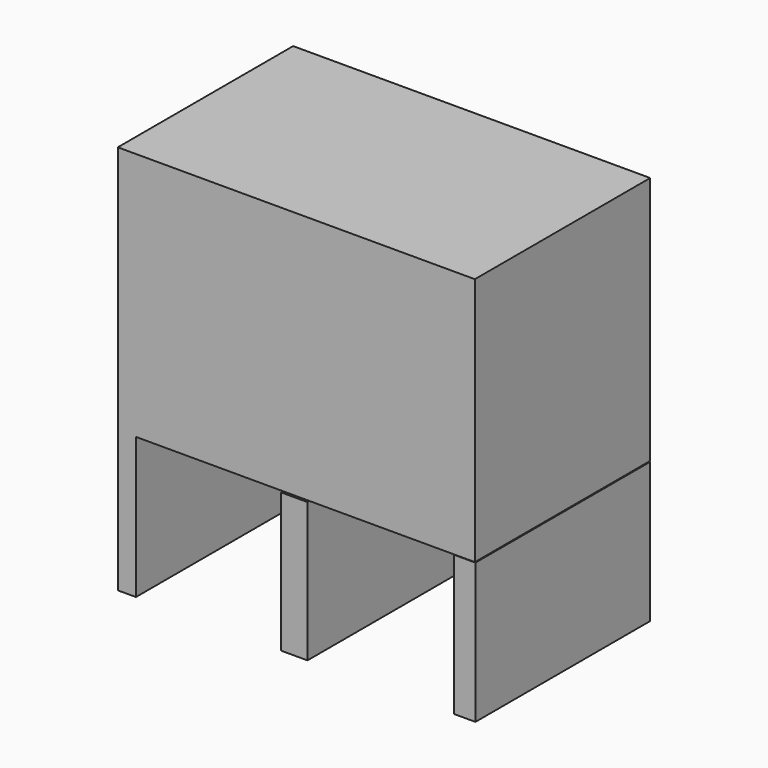
from build123d import *

# Parameters (mm, degrees)
F0_W     = 126.2088567019
F0_H     = 88.0255773664
F1_DEPTH = 77.47
F2_W     = 6.4124614
F2_H     = 49.8422943056
F4_DEPTH = 77.47
F2_W_2   = 9.3272165395
F2_H_2   = 49.2593422532
F5_DEPTH = 77.47
F2_W_3   = 7.5783729553
F2_H_3   = 49.550820142
F6_DEPTH = 77.216


# Not quite as in the source:
# - the program builds the solid bodies; features that only make, move or delete a surface that nothing else refers to are left out


with BuildPart() as f1:
    # F0 (on Front) → F1 (new body)
    with BuildSketch(Plane.XZ):
        with Locations((0.7286891341, 17.9257392883)):
            Rectangle(F0_W, F0_H)
    extrude(amount=F1_DEPTH)

    # F2 (on Front) → F4 (join)
    with BuildSketch(Plane.XZ):
        with Locations((-59.1695085168, -51.0081965476)):
            Rectangle(F2_W, F2_H)
    extrude(amount=F4_DEPTH)


with BuildPart() as f5:
    # F2 (on Front) → F5 (new body)
    with BuildSketch(Plane.XZ):
        with Locations((2.328e-07, -51.2996725738)):
            Rectangle(F2_W_2, F2_H_2)
    extrude(amount=F5_DEPTH)


with BuildPart() as f6:
    # F2 (on Front) → F6 (new body)
    with BuildSketch(Plane.XZ):
        with Locations((60.043938458, -51.1539336294)):
            Rectangle(F2_W_3, F2_H_3)
    extrude(amount=F6_DEPTH)


solid = Compound([f1.part, f5.part, f6.part])
